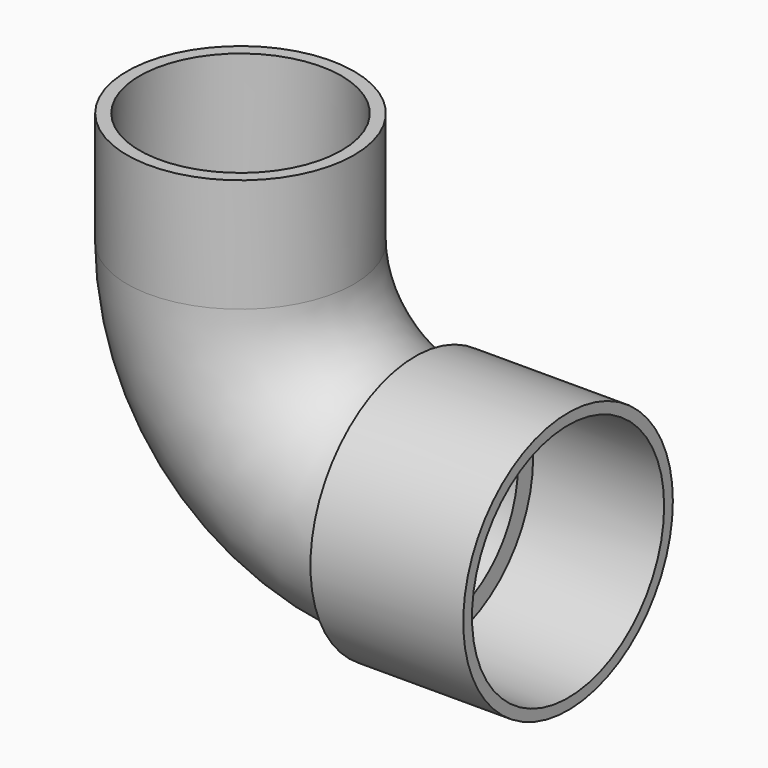
from build123d import *

# Parameters (mm, degrees)
F0_R     = 26
F0_R_2   = 23.125
F3_R     = 26
F3_R_2   = 23.125
F3_R_3   = 22.5
F4_DEPTH = 1
F5_R     = 26
F5_R_2   = 23.125
F6_DEPTH = 25
F7_R     = 27.5
F7_R_2   = 26
F7_R_3   = 23.125
F8_DEPTH = 5
F7_R_4   = 30
F9_DEPTH = 35


with BuildPart() as f2:
    # F2: sweep along a path in F1
    with BuildLine(Plane.XZ) as f2_path:
        ThreePointArc((0, 0), (11.7157287525, -28.2842712475), (40, -40))
    # F0 (on Top) → F2 (sweep)
    with BuildSketch(Plane.XY):
        Circle(F0_R)
        Circle(F0_R_2, mode=Mode.SUBTRACT)
    sweep(path=f2_path.line)

    # F3 (on face) → F4 (join)
    with BuildSketch(Plane.XY):
        Circle(F3_R)
        Circle(F3_R_2, mode=Mode.SUBTRACT)
        Circle(F3_R_2)
        Circle(F3_R_3, mode=Mode.SUBTRACT)
    extrude(amount=F4_DEPTH)

    # F5 (on face) → F6 (join)
    with BuildSketch(Plane.XY.offset(1)):
        Circle(F5_R)
        Circle(F5_R_2, mode=Mode.SUBTRACT)
    extrude(amount=F6_DEPTH)

    # F7 (on face) → F8 (join)
    with BuildSketch(Plane.YZ.offset(40)):
        with Locations((0, -40)):
            Circle(F7_R)
        with Locations((0, -40)):
            Circle(F7_R_2, mode=Mode.SUBTRACT)
        with Locations((0, -40)):
            Circle(F7_R_2)
        with Locations((0, -40)):
            Circle(F7_R_3, mode=Mode.SUBTRACT)
    extrude(amount=F8_DEPTH)

    # F7 (on face) → F9 (join)
    with BuildSketch(Plane.YZ.offset(40)):
        with Locations((0, -40)):
            Circle(F7_R_4)
        with Locations((0, -40)):
            Circle(F7_R, mode=Mode.SUBTRACT)
    extrude(amount=F9_DEPTH)


solid = f2.part
